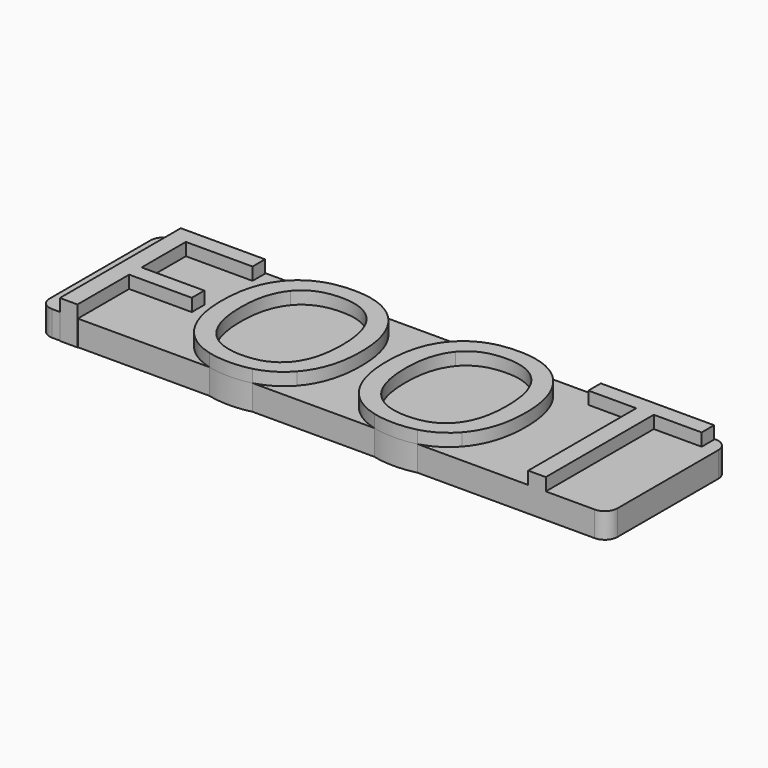
from build123d import *

# Parameters (mm, degrees)
F0_W          = 90
F0_H          = 24
F1_DEPTH      = 4
F2_R          = 2
F3_W          = 2.7838294402
F3_H          = 0.0789887575
F4_DEPTH      = 2
F4_DEPTH_BACK = 4
F5_TEXT_SIZE  = 17.3611111111
F6_DEPTH      = 1.5


# Not quite as in the source:
# - a feature names something its author has since deleted; it is built from what else it names
# - Text() gives the source's letters only with a copy of the font that has no kerning and outlines rounded to 1/6400 em; it was checked with that copy


with BuildPart() as f1:
    # F0 (on Top) → F1 (new body)
    with BuildSketch(Plane.XY):
        Rectangle(F0_W, F0_H)
    extrude(amount=F1_DEPTH)

    # F2
    f2_edges = [f1.edges().sort_by_distance(p)[0] for p in [
        (-45, -12, 2),
        (45, 12, 2),
        (-45, 12, 2),
        (45, -12, 2),
    ]]
    fillet(f2_edges, radius=F2_R)

    # F3 (on face) → F4 (join, two sides)
    with BuildSketch(Plane.XY.offset(4)) as f4_sk:
        Polygon((-41.7076367449, -12), (-38.9238073047, -12), (-38.9238073047, -1.8401584435), (-28.994291373, -1.8401584435), (-28.994291373, 0.6343566144), (-38.9238073047, 0.6343566144), (-38.9238073047, 9.4000116503), (-28.3546921419, 9.4000116503), (-28.3546921419, 11.8745267082), (-41.7076367449, 11.8745267082), align=None)
        with Locations((-40.3157220248, -12.0394943787)):
            Rectangle(F3_W, F3_H)
        with BuildLine():
            add(Edge.make_bspline(
                [(-18.049303248, -12), (-20.9050665567, -11.2582097922), (-22.7581988699, -9.1719578261)],
                knots=[0.3555611785, 0.3555611785, 0.3555611785, 1, 1, 1], degree=2))
            Line((-18.049303248, -12), (-11.2268048981, -12))
            add(Edge.make_bspline(
                [(-6.5087085688, -9.1142890429), (-8.3928948161, -11.2480026582), (-11.2268048981, -12)],
                knots=[0, 0, 0, 0.6475640702, 0.6475640702, 0.6475640702], degree=2))
            add(Edge.make_bspline(
                [(-3.599056329, -0.0681540164), (-3.599056329, -5.8193044795), (-6.5087085688, -9.1142890429)],
                knots=[0, 0, 0, 1, 1, 1], degree=2))
            add(Edge.make_bspline(
                [(-6.4982233355, 8.9753597018), (-3.599056329, 5.6987242966), (-3.599056329, -0.0681540164)],
                knots=[0, 0, 0, 1, 1, 1], degree=2))
            add(Edge.make_bspline(
                [(-11.8713930407, 12), (-8.5933918618, 11.343316897), (-6.4982233355, 8.9753597018)],
                knots=[0.2773205125, 0.2773205125, 0.2773205125, 1, 1, 1], degree=2))
            Line((-11.8713930407, 12), (-17.3406616525, 12))
            add(Edge.make_bspline(
                [(-22.750334945, 9.0330284849), (-20.6736636867, 11.3513487623), (-17.3406616525, 12)],
                knots=[0, 0, 0, 0.7202063736, 0.7202063736, 0.7202063736], degree=2))
            add(Edge.make_bspline(
                [(-25.6337741015, -0.0366983165), (-25.6337741015, 5.8140618629), (-22.750334945, 9.0330284849)],
                knots=[0, 0, 0, 1, 1, 1], degree=2))
            add(Edge.make_bspline(
                [(-22.7581988699, -9.1719578261), (-25.6337741015, -5.9346420458), (-25.6337741015, -0.0366983165)],
                knots=[0, 0, 0, 1, 1, 1], degree=2))
        make_face()
        with BuildLine():
            add(Edge.make_bspline(
                [(-22.6874235452, -0.0681540164), (-22.6874235452, -4.933302266), (-20.6139686608, -7.4497582571)],
                knots=[0, 0, 0, 1, 1, 1], degree=2))
            add(Edge.make_bspline(
                [(-20.6139686608, 7.2452962078), (-22.6874235452, 4.7288402167), (-22.6874235452, -0.0681540164)],
                knots=[0, 0, 0, 1, 1, 1], degree=2))
            add(Edge.make_bspline(
                [(-14.5613677404, 9.761752199), (-18.5405137764, 9.761752199), (-20.6139686608, 7.2452962078)],
                knots=[0, 0, 0, 1, 1, 1], degree=2))
            add(Edge.make_bspline(
                [(-8.5742995282, 7.2636453661), (-10.5979495544, 9.761752199), (-14.5613677404, 9.761752199)],
                knots=[0, 0, 0, 1, 1, 1], degree=2))
            add(Edge.make_bspline(
                [(-6.550649502, -0.0681540164), (-6.550649502, 4.7655385332), (-8.5742995282, 7.2636453661)],
                knots=[0, 0, 0, 1, 1, 1], degree=2))
            add(Edge.make_bspline(
                [(-8.5821634531, -7.4602434904), (-6.550649502, -4.9542727326), (-6.550649502, -0.0681540164)],
                knots=[0, 0, 0, 1, 1, 1], degree=2))
            add(Edge.make_bspline(
                [(-14.5928234403, -9.9662142483), (-10.6136774043, -9.9662142483), (-8.5821634531, -7.4602434904)],
                knots=[0, 0, 0, 1, 1, 1], degree=2))
            add(Edge.make_bspline(
                [(-20.6139686608, -7.4497582571), (-18.5405137764, -9.9662142483), (-14.5928234403, -9.9662142483)],
                knots=[0, 0, 0, 1, 1, 1], degree=2))
        make_face(mode=Mode.SUBTRACT)
        with BuildLine():
            Line((-11.2268048981, -12), (-18.049303248, -12))
            add(Edge.make_bspline(
                [(-14.5928234403, -12.4092736063), (-16.473671033, -12.4092736063), (-18.049303248, -12)],
                knots=[0, 0, 0, 0.3555611785, 0.3555611785, 0.3555611785], degree=2))
            add(Edge.make_bspline(
                [(-11.2268048981, -12), (-12.7691568916, -12.4092736063), (-14.5928234403, -12.4092736063)],
                knots=[0.6475640702, 0.6475640702, 0.6475640702, 1, 1, 1], degree=2))
        make_face()
        with BuildLine():
            Line((14.9023964766, -12), (8.0798981267, -12))
            add(Edge.make_bspline(
                [(11.5363779344, -12.4092736063), (9.6555303417, -12.4092736063), (8.0798981267, -12)],
                knots=[0, 0, 0, 0.3555611785, 0.3555611785, 0.3555611785], degree=2))
            add(Edge.make_bspline(
                [(14.9023964766, -12), (13.3600444831, -12.4092736063), (11.5363779344, -12.4092736063)],
                knots=[0.6475640702, 0.6475640702, 0.6475640702, 1, 1, 1], degree=2))
        make_face()
        with BuildLine():
            add(Edge.make_bspline(
                [(8.0798981267, -12), (5.224134818, -11.2582097922), (3.3710025048, -9.1719578261)],
                knots=[0.3555611785, 0.3555611785, 0.3555611785, 1, 1, 1], degree=2))
            Line((8.0798981267, -12), (14.9023964766, -12))
            add(Edge.make_bspline(
                [(19.620492806, -9.1142890429), (17.7363065586, -11.2480026582), (14.9023964766, -12)],
                knots=[0, 0, 0, 0.6475640702, 0.6475640702, 0.6475640702], degree=2))
            add(Edge.make_bspline(
                [(22.5301450457, -0.0681540164), (22.5301450457, -5.8193044795), (19.620492806, -9.1142890429)],
                knots=[0, 0, 0, 1, 1, 1], degree=2))
            add(Edge.make_bspline(
                [(19.6309780393, 8.9753597018), (22.5301450457, 5.6987242966), (22.5301450457, -0.0681540164)],
                knots=[0, 0, 0, 1, 1, 1], degree=2))
            add(Edge.make_bspline(
                [(14.257808334, 12), (17.5358095129, 11.343316897), (19.6309780393, 8.9753597018)],
                knots=[0.2773205125, 0.2773205125, 0.2773205125, 1, 1, 1], degree=2))
            Line((14.257808334, 12), (8.7885397222, 12))
            add(Edge.make_bspline(
                [(3.3788664298, 9.0330284849), (5.4555376881, 11.3513487623), (8.7885397222, 12)],
                knots=[0, 0, 0, 0.7202063736, 0.7202063736, 0.7202063736], degree=2))
            add(Edge.make_bspline(
                [(0.4954272733, -0.0366983165), (0.4954272733, 5.8140618629), (3.3788664298, 9.0330284849)],
                knots=[0, 0, 0, 1, 1, 1], degree=2))
            add(Edge.make_bspline(
                [(3.3710025048, -9.1719578261), (0.4954272733, -5.9346420458), (0.4954272733, -0.0366983165)],
                knots=[0, 0, 0, 1, 1, 1], degree=2))
        make_face()
        with BuildLine():
            add(Edge.make_bspline(
                [(3.4417778296, -0.0681540164), (3.4417778296, -4.933302266), (5.5152327139, -7.4497582571)],
                knots=[0, 0, 0, 1, 1, 1], degree=2))
            add(Edge.make_bspline(
                [(5.5152327139, 7.2452962078), (3.4417778296, 4.7288402167), (3.4417778296, -0.0681540164)],
                knots=[0, 0, 0, 1, 1, 1], degree=2))
            add(Edge.make_bspline(
                [(11.5678336343, 9.761752199), (7.5886875983, 9.761752199), (5.5152327139, 7.2452962078)],
                knots=[0, 0, 0, 1, 1, 1], degree=2))
            add(Edge.make_bspline(
                [(17.5549018466, 7.2636453661), (15.5312518204, 9.761752199), (11.5678336343, 9.761752199)],
                knots=[0, 0, 0, 1, 1, 1], degree=2))
            add(Edge.make_bspline(
                [(19.5785518728, -0.0681540164), (19.5785518728, 4.7655385332), (17.5549018466, 7.2636453661)],
                knots=[0, 0, 0, 1, 1, 1], degree=2))
            add(Edge.make_bspline(
                [(17.5470379216, -7.4602434904), (19.5785518728, -4.9542727326), (19.5785518728, -0.0681540164)],
                knots=[0, 0, 0, 1, 1, 1], degree=2))
            add(Edge.make_bspline(
                [(11.5363779344, -9.9662142483), (15.5155239704, -9.9662142483), (17.5470379216, -7.4602434904)],
                knots=[0, 0, 0, 1, 1, 1], degree=2))
            add(Edge.make_bspline(
                [(5.5152327139, -7.4497582571), (7.5886875983, -9.9662142483), (11.5363779344, -9.9662142483)],
                knots=[0, 0, 0, 1, 1, 1], degree=2))
        make_face(mode=Mode.SUBTRACT)
        with BuildLine():
            add(Edge.make_bspline(
                [(-17.3406616525, 12), (-16.0458206732, 12.2519951069), (-14.5613677404, 12.2519951069)],
                knots=[0.7202063736, 0.7202063736, 0.7202063736, 1, 1, 1], degree=2))
            Line((-17.3406616525, 12), (-11.8713930407, 12))
            add(Edge.make_bspline(
                [(-14.5613677404, 12.2519951069), (-13.1292908816, 12.2519951069), (-11.8713930407, 12)],
                knots=[0, 0, 0, 0.2773205125, 0.2773205125, 0.2773205125], degree=2))
        make_face()
        with BuildLine():
            add(Edge.make_bspline(
                [(8.7885397222, 12), (10.0833807016, 12.2519951069), (11.5678336343, 12.2519951069)],
                knots=[0.7202063736, 0.7202063736, 0.7202063736, 1, 1, 1], degree=2))
            Line((8.7885397222, 12), (14.257808334, 12))
            add(Edge.make_bspline(
                [(11.5678336343, 12.2519951069), (12.9999104931, 12.2519951069), (14.257808334, 12)],
                knots=[0, 0, 0, 0.2773205125, 0.2773205125, 0.2773205125], degree=2))
        make_face()
        Polygon((32.4544183608, 9.4000116503), (32.4544183608, -12), (35.238247801, -12), (35.238247801, 9.4000116503), (42.824314091, 9.4000116503), (42.824314091, 11.8745267082), (24.8683520708, 11.8745267082), (24.8683520708, 9.4000116503), align=None)
    extrude(amount=F4_DEPTH)
    extrude(f4_sk.sketch, amount=-F4_DEPTH_BACK)

    # F5 (on face) → F6 (cut)
    with BuildSketch(Plane(origin=(0, 0, 0), x_dir=(1, 0, 0), z_dir=(0, 0, -1))):
        with Locations((-38.3409288194, -6.25)):
            Text('12 inches', F5_TEXT_SIZE, font='Open Sans', text_align=(TextAlign.LEFT, TextAlign.BOTTOM))
    extrude(amount=-F6_DEPTH, mode=Mode.SUBTRACT)


solid = f1.part
